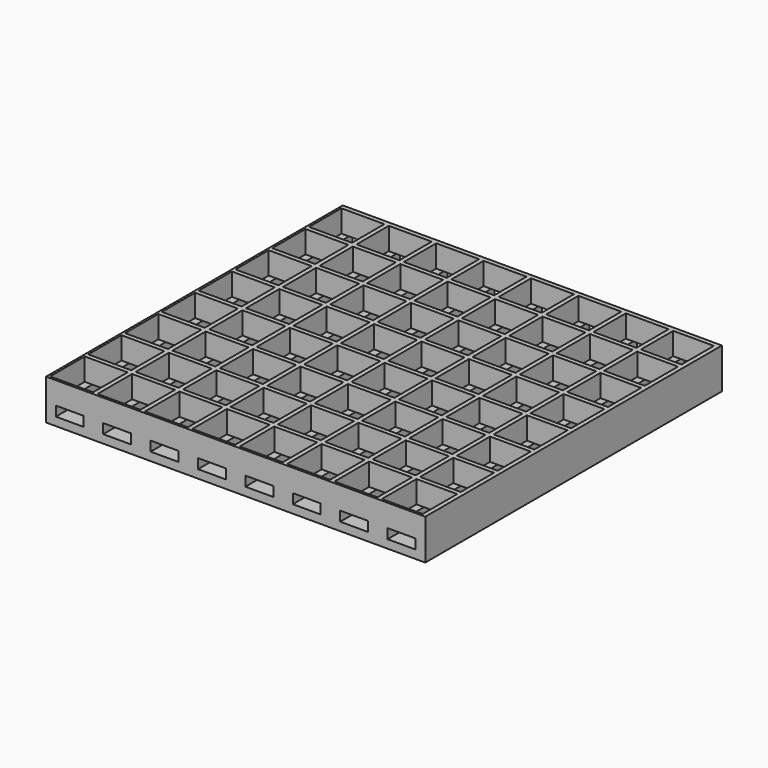
from build123d import *

# Parameters (mm, degrees)
F0_W                 = 3.5
F0_H                 = 3.5
F0_W_2               = 7
F1_DEPTH             = 133
F2_W                 = 0.8
F2_H                 = 8
F2_W_2               = 1.6
F3_DEPTH             = 133
F4_W                 = 1.6
F4_H                 = 8
F4_W_2               = 0.8
F5_DEPTH             = 136
F8_D                 = 3.5
F8_DEPTH             = 12
F8_CSINK_D           = 6.5
F8_CSINK_ANGLE       = 90
F8_TIP               = 1.0515060833
F8_ON_F6_D           = 3.5
F8_ON_F6_DEPTH       = 12
F8_ON_F6_CSINK_D     = 6.5
F8_ON_F6_CSINK_ANGLE = 90
F8_ON_F6_TIP         = 1.0515060833


# Not quite as in the source:
# - a feature names something its author has since deleted; it is built from what else it names


with BuildPart() as f1:
    # F0 (on Front) → F1 (new body)
    with BuildSketch(Plane.XZ):
        with Locations((-66.25, 4.75)):
            Rectangle(F0_W, F0_H)
        with Locations((-17, 4.75)):
            Rectangle(F0_W_2, F0_H)
        with Locations((66.25, 4.75)):
            Rectangle(F0_W, F0_H)
        Polygon((-64.5, 3), (-68, 3), (-68, 0), (68, 0), (68, 3), (64.5, 3), (54.5, 3), (47.5, 3), (37.5, 3), (30.5, 3), (20.5, 3), (13.5, 3), (3.5, 3), (-3.5, 3), (-13.5, 3), (-20.5, 3), (-30.5, 3), (-37.5, 3), (-47.5, 3), (-54.5, 3), align=None)
        with Locations((-51, 4.75)):
            Rectangle(F0_W_2, F0_H)
        with Locations((-34, 4.75)):
            Rectangle(F0_W_2, F0_H)
        with Locations((0, 4.75)):
            Rectangle(F0_W_2, F0_H)
        with Locations((17, 4.75)):
            Rectangle(F0_W_2, F0_H)
        with Locations((34, 4.75)):
            Rectangle(F0_W_2, F0_H)
        with Locations((51, 4.75)):
            Rectangle(F0_W_2, F0_H)
    extrude(amount=F1_DEPTH)

    # F2 (on face) → F3 (join, through all)
    with BuildSketch(Plane.XZ.offset(133)):
        with Locations((-67.6, 10.5)):
            Rectangle(F2_W, F2_H)
        with Locations((-51, 10.5)):
            Rectangle(F2_W_2, F2_H)
        with Locations((-34, 10.5)):
            Rectangle(F2_W_2, F2_H)
        with Locations((-17, 10.5)):
            Rectangle(F2_W_2, F2_H)
        with Locations((0, 10.5)):
            Rectangle(F2_W_2, F2_H)
        with Locations((17, 10.5)):
            Rectangle(F2_W_2, F2_H)
        with Locations((34, 10.5)):
            Rectangle(F2_W_2, F2_H)
        with Locations((51, 10.5)):
            Rectangle(F2_W_2, F2_H)
        with Locations((67.2, 10.5)):
            Rectangle(F2_W_2, F2_H)
    extrude(amount=-F3_DEPTH)

    # F4 (on face) → F5 (join, through all)
    with BuildSketch(Plane(origin=(-68, 0, 0), x_dir=(0, -1, 0), z_dir=(-1, 0, 0))):
        with Locations((0.8, 10.5)):
            Rectangle(F4_W, F4_H)
        with Locations((16.9, 10.5)):
            Rectangle(F4_W, F4_H)
        with Locations((33.4, 10.5)):
            Rectangle(F4_W, F4_H)
        with Locations((49.9, 10.5)):
            Rectangle(F4_W, F4_H)
        with Locations((66.4, 10.5)):
            Rectangle(F4_W, F4_H)
        with Locations((82.9, 10.5)):
            Rectangle(F4_W, F4_H)
        with Locations((99.4, 10.5)):
            Rectangle(F4_W, F4_H)
        with Locations((115.9, 10.5)):
            Rectangle(F4_W, F4_H)
        with Locations((132.6, 10.5)):
            Rectangle(F4_W_2, F4_H)
    extrude(amount=-F5_DEPTH)

    # F8
    with Locations(Plane.XY.offset(3)):
        with Locations((42.5, -42), (42.5, -91)):
            CounterSinkHole(F8_D / 2, F8_CSINK_D / 2, depth=F8_DEPTH, counter_sink_angle=F8_CSINK_ANGLE)
            with Locations((0, 0, -(F8_DEPTH + F8_TIP / 2))):  # 118° drill point
                Cone(0, F8_D / 2, F8_TIP, mode=Mode.SUBTRACT)

    # F8 on F6
    with Locations(Plane.XY.offset(3)):
        with Locations((-42.5, -42), (-42.5, -91)):
            CounterSinkHole(F8_ON_F6_D / 2, F8_ON_F6_CSINK_D / 2, depth=F8_ON_F6_DEPTH, counter_sink_angle=F8_ON_F6_CSINK_ANGLE)
            with Locations((0, 0, -(F8_ON_F6_DEPTH + F8_ON_F6_TIP / 2))):  # 118° drill point
                Cone(0, F8_ON_F6_D / 2, F8_ON_F6_TIP, mode=Mode.SUBTRACT)


solid = f1.part
